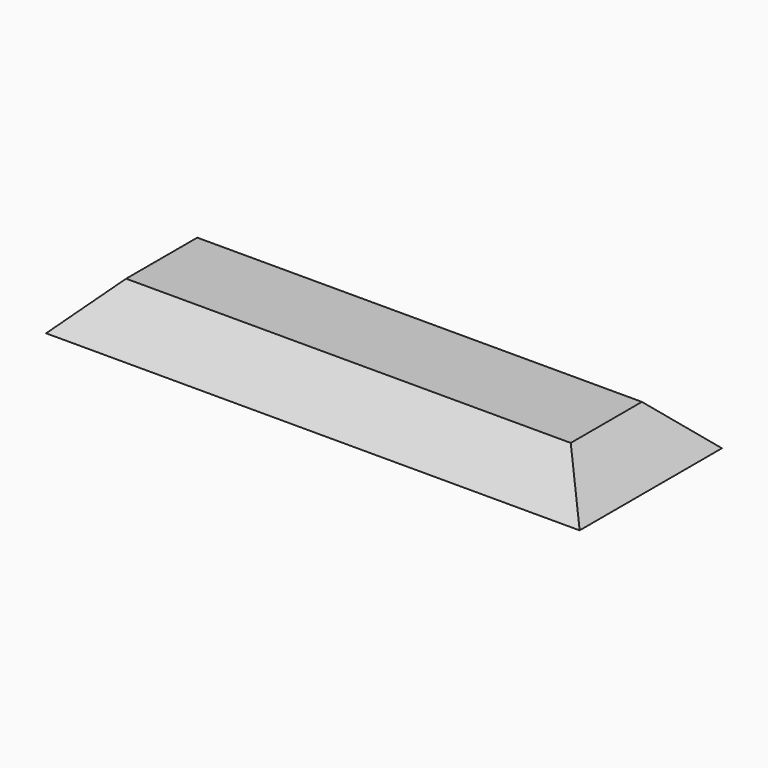
from build123d import *

# Parameters (mm, degrees)
F0_W     = 50.8
F0_H     = 12.7
F1_DEPTH = 76.2
F2_SIZE  = 12.69999


# Not quite as in the source:
# - a fillet or chamfer is up to 0.001 mm smaller than in the source, because OpenCascade refuses the exact size


with BuildPart() as f1:
    # F0 (on Right) → F1 (new body, symmetric)
    with BuildSketch(Plane.YZ):
        Rectangle(F0_W, F0_H)
    extrude(amount=F1_DEPTH, both=True)

    # F2 (size 12.7 in the source; OpenCascade refuses exactly that, so slightly less here)
    f2_edges = [f1.edges().sort_by_distance(p)[0] for p in [
        (0, 25.4, 6.35),
        (-76.2, 0, 6.35),
        (0, -25.4, 6.35),
        (76.2, 0, 6.35),
    ]]
    chamfer(f2_edges, length=F2_SIZE)


solid = f1.part
